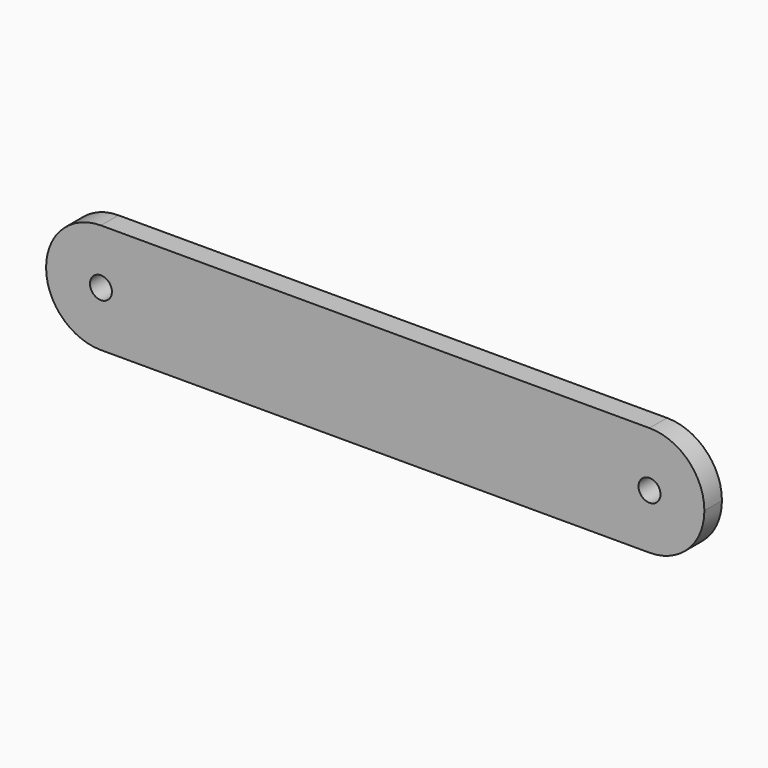
from build123d import *

# Parameters (mm, degrees)
F0_W     = 60
F0_H     = 10
F0_R     = 1
F1_DEPTH = 2
F2_R     = 4.99999


# Not quite as in the source:
# - a fillet or chamfer is up to 0.001 mm smaller than in the source, because OpenCascade refuses the exact size


with BuildPart() as f1:
    # F0 (on Front) → F1 (new body)
    with BuildSketch(Plane.XZ):
        with Locations((30, -5)):
            Rectangle(F0_W, F0_H)
        with Locations((5, -5)):
            Circle(F0_R, mode=Mode.SUBTRACT)
        with Locations((55, -5)):
            Circle(F0_R, mode=Mode.SUBTRACT)
    extrude(amount=F1_DEPTH)

    # F2 (radius 5 in the source; OpenCascade refuses exactly that, so slightly less here)
    f2_edges = [f1.edges().sort_by_distance(p)[0] for p in [
        (0, -1, 0),
        (0, -1, -10),
        (60, -1, 0),
        (60, -1, -10),
    ]]
    fillet(f2_edges, radius=F2_R)


solid = f1.part
